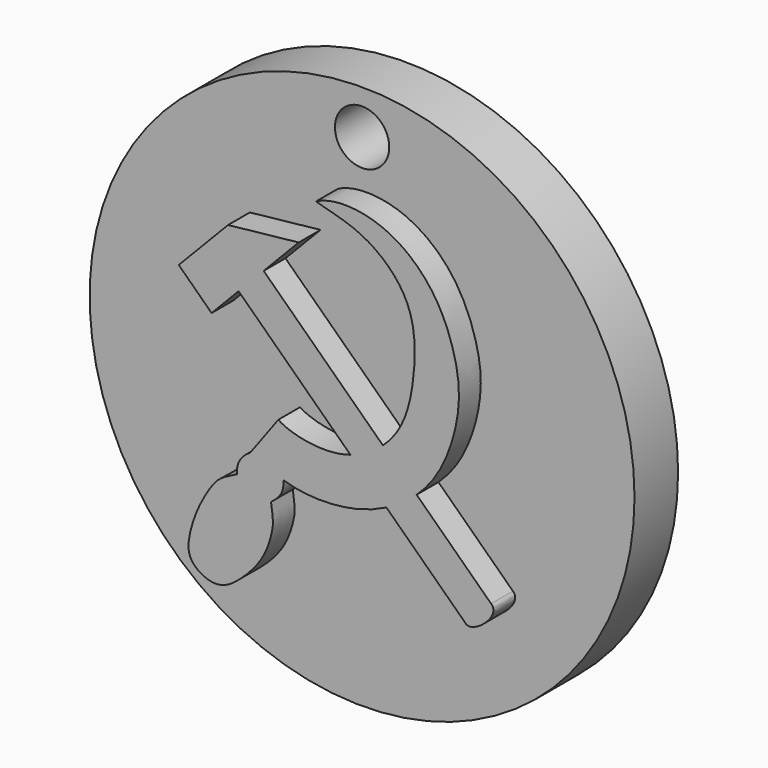
from build123d import *

# Parameters (mm, degrees)
F0_R     = 12.7
F0_R_2   = 1.2657765137
F1_DEPTH = 2.54
F2_DEPTH = 3.81


with BuildPart() as f1:
    # F0 (on Front) → F1 (new body)
    with BuildSketch(Plane.XZ):
        Circle(F0_R)
        with BuildLine():
            Line((-5.9980981207, 1.9931174991), (-7.5295561864, 3.4678540847))
            Line((-7.5295561864, 3.4678540847), (-5.2310121246, 5.8548050001))
            Line((-5.2310121246, 5.8548050001), (-1.9379338482, 6.2094442546))
            Line((-1.9379338482, 6.2094442546), (-3.5720530129, 4.5124734196))
            Line((-3.5720530129, 4.5124734196), (1.9898101435, -0.8433918597))
            add(Edge.make_bspline(
                [(1.9898101435, -0.8433918597), (2.181839817, -0.6686980904), (2.9923268789, 0.2254004935), (3.5097247457, 2.2611806235), (3.5582576463, 5.5722342669), (1.0757347307, 7.7154267447), (-0.6801631143, 8.0019912543), (-1.1338472479, 8.1532060726)],
                knots=[0.2966989611, 0.2966989611, 0.2966989611, 0.2966989611, 0.3408733214, 0.5050447961, 0.6807588711, 0.8554095009, 1, 1, 1, 1], degree=3))
            add(Edge.make_bspline(
                [(-1.1338472479, 8.1532060726), (-0.3417312748, 8.5800115317), (2.0076237784, 8.4565524057), (4.3362523203, 6.5122135204), (5.3334470637, 4.2153426842), (5.7115580421, 1.9856279561), (4.9509483833, -0.7254500645), (4.0310276615, -1.9202184076), (3.5599331607, -2.3553613411)],
                knots=[0, 0, 0, 0, 0.1298019735, 0.2598346579, 0.3771771158, 0.4898846412, 0.6185830731, 0.71201256, 0.71201256, 0.71201256, 0.71201256], degree=3))
            Line((3.5599331607, -2.3553613411), (7.0293718017, -5.6963004173))
            add(Edge.make_bspline(
                [(7.0293718017, -5.6963004173), (7.5221849988, -6.1239386803), (6.1995871365, -7.1983786766), (5.8641284704, -6.9122067653)],
                knots=[0, 0, 0, 0, 1.6841081521, 1.6841081521, 1.6841081521, 1.6841081521], degree=3))
            Line((5.8641284704, -6.9122067653), (2.1508335508, -3.3364432536))
            add(Edge.make_bspline(
                [(2.1508335508, -3.3364432536), (1.6752853418, -3.5797182972), (0.1572248048, -4.1350575123), (-1.7609307542, -4.0777400136), (-2.6475286577, -3.7737630773)],
                knots=[0.7925286484, 0.7925286484, 0.7925286484, 0.7925286484, 0.8643366586, 1, 1, 1, 1], degree=3))
            add(Edge.make_bspline(
                [(-2.6475286577, -3.7737630773), (-2.6181081776, -4.3935817666), (-2.9226117767, -4.6085258946), (-3.22854775, -4.8588160425)],
                knots=[0, 0, 0, 0, 1.230822133, 1.230822133, 1.230822133, 1.230822133], degree=3))
            add(Edge.make_bspline(
                [(-4.8033702187, -4.2323740199), (-5.4212825728, -4.5293064688), (-5.8316147769, -4.7778373261), (-6.6343124935, -6.1229466147), (-7.0458907635, -7.3455408415), (-7.16887863, -8.5506128462), (-5.7407828877, -9.3119682828), (-4.6015383692, -8.4966283885), (-3.5049723158, -7.3084696393), (-3.0930861156, -5.8275163642), (-3.1405196662, -5.4844899198), (-3.22854775, -4.8588160425)],
                knots=[0, 0, 0, 0, 0.1093958452, 0.2246343447, 0.3382227988, 0.4386314231, 0.5491357113, 0.6596208576, 0.7857586816, 0.8981987194, 1, 1, 1, 1], degree=3))
            add(Edge.make_bspline(
                [(-4.1932296008, -3.1469750684), (-4.7146673314, -3.4729705658), (-4.8571061343, -3.8741342723), (-4.8033702187, -4.2323740199)],
                knots=[0, 0, 0, 0, 1.2451355178, 1.2451355178, 1.2451355178, 1.2451355178], degree=3))
            Line((-4.1932296008, -3.1469750684), (-2.8876534512, -1.373414264))
            add(Edge.make_bspline(
                [(-2.8876534512, -1.373414264), (-2.386986779, -1.7200056059), (-0.9613233884, -2.068928273), (0.2712498796, -1.7849151458), (0.4732034023, -1.7209484435)],
                knots=[0, 0, 0, 0, 0.1659033418, 0.1998088447, 0.1998088447, 0.1998088447, 0.1998088447], degree=3))
            Line((0.4732034023, -1.7209484435), (-4.740216914, 3.2993794706))
            Line((-4.740216914, 3.2993794706), (-5.9980981207, 1.9931174991))
        make_face(mode=Mode.SUBTRACT)
        with Locations((0, 10.6459101662)):
            Circle(F0_R_2, mode=Mode.SUBTRACT)
        with BuildLine():
            add(Edge.make_bspline(
                [(0.4732034023, -1.7209484435), (1.0503162203, -1.5381538908), (1.5686206286, -1.2265575579), (1.9898101435, -0.8433918597)],
                knots=[0.1998088447, 0.1998088447, 0.1998088447, 0.1998088447, 0.2966989611, 0.2966989611, 0.2966989611, 0.2966989611], degree=3))
            add(Edge.make_bspline(
                [(-2.8876534512, -1.373414264), (-2.386986779, -1.7200056059), (-0.9613233884, -2.068928273), (0.2712498796, -1.7849151458), (0.4732034023, -1.7209484435)],
                knots=[0, 0, 0, 0, 0.1659033418, 0.1998088447, 0.1998088447, 0.1998088447, 0.1998088447], degree=3))
            Line((-2.8876534512, -1.373414264), (-4.1932296008, -3.1469750684))
            add(Edge.make_bspline(
                [(-4.1932296008, -3.1469750684), (-4.7146673314, -3.4729705658), (-4.8571061343, -3.8741342723), (-4.8033702187, -4.2323740199)],
                knots=[0, 0, 0, 0, 1.2451355178, 1.2451355178, 1.2451355178, 1.2451355178], degree=3))
            add(Edge.make_bspline(
                [(-4.8033702187, -4.2323740199), (-5.4212825728, -4.5293064688), (-5.8316147769, -4.7778373261), (-6.6343124935, -6.1229466147), (-7.0458907635, -7.3455408415), (-7.16887863, -8.5506128462), (-5.7407828877, -9.3119682828), (-4.6015383692, -8.4966283885), (-3.5049723158, -7.3084696393), (-3.0930861156, -5.8275163642), (-3.1405196662, -5.4844899198), (-3.22854775, -4.8588160425)],
                knots=[0, 0, 0, 0, 0.1093958452, 0.2246343447, 0.3382227988, 0.4386314231, 0.5491357113, 0.6596208576, 0.7857586816, 0.8981987194, 1, 1, 1, 1], degree=3))
            add(Edge.make_bspline(
                [(-2.6475286577, -3.7737630773), (-2.6181081776, -4.3935817666), (-2.9226117767, -4.6085258946), (-3.22854775, -4.8588160425)],
                knots=[0, 0, 0, 0, 1.230822133, 1.230822133, 1.230822133, 1.230822133], degree=3))
            add(Edge.make_bspline(
                [(2.1508335508, -3.3364432536), (1.6752853418, -3.5797182972), (0.1572248048, -4.1350575123), (-1.7609307542, -4.0777400136), (-2.6475286577, -3.7737630773)],
                knots=[0.7925286484, 0.7925286484, 0.7925286484, 0.7925286484, 0.8643366586, 1, 1, 1, 1], degree=3))
            add(Edge.make_bspline(
                [(3.5599331607, -2.3553613411), (3.4359379602, -2.4698938503), (3.0108649417, -2.8296074096), (2.5211954544, -3.1469781131), (2.1508335508, -3.3364432536)],
                knots=[0.71201256, 0.71201256, 0.71201256, 0.71201256, 0.7366038212, 0.7925286484, 0.7925286484, 0.7925286484, 0.7925286484], degree=3))
            add(Edge.make_bspline(
                [(-1.1338472479, 8.1532060726), (-0.3417312748, 8.5800115317), (2.0076237784, 8.4565524057), (4.3362523203, 6.5122135204), (5.3334470637, 4.2153426842), (5.7115580421, 1.9856279561), (4.9509483833, -0.7254500645), (4.0310276615, -1.9202184076), (3.5599331607, -2.3553613411)],
                knots=[0, 0, 0, 0, 0.1298019735, 0.2598346579, 0.3771771158, 0.4898846412, 0.6185830731, 0.71201256, 0.71201256, 0.71201256, 0.71201256], degree=3))
            add(Edge.make_bspline(
                [(1.9898101435, -0.8433918597), (2.181839817, -0.6686980904), (2.9923268789, 0.2254004935), (3.5097247457, 2.2611806235), (3.5582576463, 5.5722342669), (1.0757347307, 7.7154267447), (-0.6801631143, 8.0019912543), (-1.1338472479, 8.1532060726)],
                knots=[0.2966989611, 0.2966989611, 0.2966989611, 0.2966989611, 0.3408733214, 0.5050447961, 0.6807588711, 0.8554095009, 1, 1, 1, 1], degree=3))
        make_face()
        with BuildLine():
            Line((7.0293718017, -5.6963004173), (3.5599331607, -2.3553613411))
            add(Edge.make_bspline(
                [(3.5599331607, -2.3553613411), (3.4359379602, -2.4698938503), (3.0108649417, -2.8296074096), (2.5211954544, -3.1469781131), (2.1508335508, -3.3364432536)],
                knots=[0.71201256, 0.71201256, 0.71201256, 0.71201256, 0.7366038212, 0.7925286484, 0.7925286484, 0.7925286484, 0.7925286484], degree=3))
            Line((2.1508335508, -3.3364432536), (5.8641284704, -6.9122067653))
            add(Edge.make_bspline(
                [(7.0293718017, -5.6963004173), (7.5221849988, -6.1239386803), (6.1995871365, -7.1983786766), (5.8641284704, -6.9122067653)],
                knots=[0, 0, 0, 0, 1.6841081521, 1.6841081521, 1.6841081521, 1.6841081521], degree=3))
        make_face()
    extrude(amount=F1_DEPTH)

    # F0 (on Front) → F2 (join)
    with BuildSketch(Plane.XZ):
        with BuildLine():
            Line((-5.2310121246, 5.8548050001), (-7.5295561864, 3.4678540847))
            Line((-7.5295561864, 3.4678540847), (-5.9980981207, 1.9931174991))
            Line((-5.9980981207, 1.9931174991), (-4.740216914, 3.2993794706))
            Line((-4.740216914, 3.2993794706), (0.4732034023, -1.7209484435))
            add(Edge.make_bspline(
                [(0.4732034023, -1.7209484435), (1.0503162203, -1.5381538908), (1.5686206286, -1.2265575579), (1.9898101435, -0.8433918597)],
                knots=[0.1998088447, 0.1998088447, 0.1998088447, 0.1998088447, 0.2966989611, 0.2966989611, 0.2966989611, 0.2966989611], degree=3))
            Line((1.9898101435, -0.8433918597), (-3.5720530129, 4.5124734196))
            Line((-3.5720530129, 4.5124734196), (-1.9379338482, 6.2094442546))
            Line((-1.9379338482, 6.2094442546), (-5.2310121246, 5.8548050001))
        make_face()
        with BuildLine():
            add(Edge.make_bspline(
                [(0.4732034023, -1.7209484435), (1.0503162203, -1.5381538908), (1.5686206286, -1.2265575579), (1.9898101435, -0.8433918597)],
                knots=[0.1998088447, 0.1998088447, 0.1998088447, 0.1998088447, 0.2966989611, 0.2966989611, 0.2966989611, 0.2966989611], degree=3))
            add(Edge.make_bspline(
                [(-2.8876534512, -1.373414264), (-2.386986779, -1.7200056059), (-0.9613233884, -2.068928273), (0.2712498796, -1.7849151458), (0.4732034023, -1.7209484435)],
                knots=[0, 0, 0, 0, 0.1659033418, 0.1998088447, 0.1998088447, 0.1998088447, 0.1998088447], degree=3))
            Line((-2.8876534512, -1.373414264), (-4.1932296008, -3.1469750684))
            add(Edge.make_bspline(
                [(-4.1932296008, -3.1469750684), (-4.7146673314, -3.4729705658), (-4.8571061343, -3.8741342723), (-4.8033702187, -4.2323740199)],
                knots=[0, 0, 0, 0, 1.2451355178, 1.2451355178, 1.2451355178, 1.2451355178], degree=3))
            add(Edge.make_bspline(
                [(-4.8033702187, -4.2323740199), (-5.4212825728, -4.5293064688), (-5.8316147769, -4.7778373261), (-6.6343124935, -6.1229466147), (-7.0458907635, -7.3455408415), (-7.16887863, -8.5506128462), (-5.7407828877, -9.3119682828), (-4.6015383692, -8.4966283885), (-3.5049723158, -7.3084696393), (-3.0930861156, -5.8275163642), (-3.1405196662, -5.4844899198), (-3.22854775, -4.8588160425)],
                knots=[0, 0, 0, 0, 0.1093958452, 0.2246343447, 0.3382227988, 0.4386314231, 0.5491357113, 0.6596208576, 0.7857586816, 0.8981987194, 1, 1, 1, 1], degree=3))
            add(Edge.make_bspline(
                [(-2.6475286577, -3.7737630773), (-2.6181081776, -4.3935817666), (-2.9226117767, -4.6085258946), (-3.22854775, -4.8588160425)],
                knots=[0, 0, 0, 0, 1.230822133, 1.230822133, 1.230822133, 1.230822133], degree=3))
            add(Edge.make_bspline(
                [(2.1508335508, -3.3364432536), (1.6752853418, -3.5797182972), (0.1572248048, -4.1350575123), (-1.7609307542, -4.0777400136), (-2.6475286577, -3.7737630773)],
                knots=[0.7925286484, 0.7925286484, 0.7925286484, 0.7925286484, 0.8643366586, 1, 1, 1, 1], degree=3))
            add(Edge.make_bspline(
                [(3.5599331607, -2.3553613411), (3.4359379602, -2.4698938503), (3.0108649417, -2.8296074096), (2.5211954544, -3.1469781131), (2.1508335508, -3.3364432536)],
                knots=[0.71201256, 0.71201256, 0.71201256, 0.71201256, 0.7366038212, 0.7925286484, 0.7925286484, 0.7925286484, 0.7925286484], degree=3))
            add(Edge.make_bspline(
                [(-1.1338472479, 8.1532060726), (-0.3417312748, 8.5800115317), (2.0076237784, 8.4565524057), (4.3362523203, 6.5122135204), (5.3334470637, 4.2153426842), (5.7115580421, 1.9856279561), (4.9509483833, -0.7254500645), (4.0310276615, -1.9202184076), (3.5599331607, -2.3553613411)],
                knots=[0, 0, 0, 0, 0.1298019735, 0.2598346579, 0.3771771158, 0.4898846412, 0.6185830731, 0.71201256, 0.71201256, 0.71201256, 0.71201256], degree=3))
            add(Edge.make_bspline(
                [(1.9898101435, -0.8433918597), (2.181839817, -0.6686980904), (2.9923268789, 0.2254004935), (3.5097247457, 2.2611806235), (3.5582576463, 5.5722342669), (1.0757347307, 7.7154267447), (-0.6801631143, 8.0019912543), (-1.1338472479, 8.1532060726)],
                knots=[0.2966989611, 0.2966989611, 0.2966989611, 0.2966989611, 0.3408733214, 0.5050447961, 0.6807588711, 0.8554095009, 1, 1, 1, 1], degree=3))
        make_face()
        with BuildLine():
            Line((7.0293718017, -5.6963004173), (3.5599331607, -2.3553613411))
            add(Edge.make_bspline(
                [(3.5599331607, -2.3553613411), (3.4359379602, -2.4698938503), (3.0108649417, -2.8296074096), (2.5211954544, -3.1469781131), (2.1508335508, -3.3364432536)],
                knots=[0.71201256, 0.71201256, 0.71201256, 0.71201256, 0.7366038212, 0.7925286484, 0.7925286484, 0.7925286484, 0.7925286484], degree=3))
            Line((2.1508335508, -3.3364432536), (5.8641284704, -6.9122067653))
            add(Edge.make_bspline(
                [(7.0293718017, -5.6963004173), (7.5221849988, -6.1239386803), (6.1995871365, -7.1983786766), (5.8641284704, -6.9122067653)],
                knots=[0, 0, 0, 0, 1.6841081521, 1.6841081521, 1.6841081521, 1.6841081521], degree=3))
        make_face()
    extrude(amount=F2_DEPTH)


solid = f1.part
